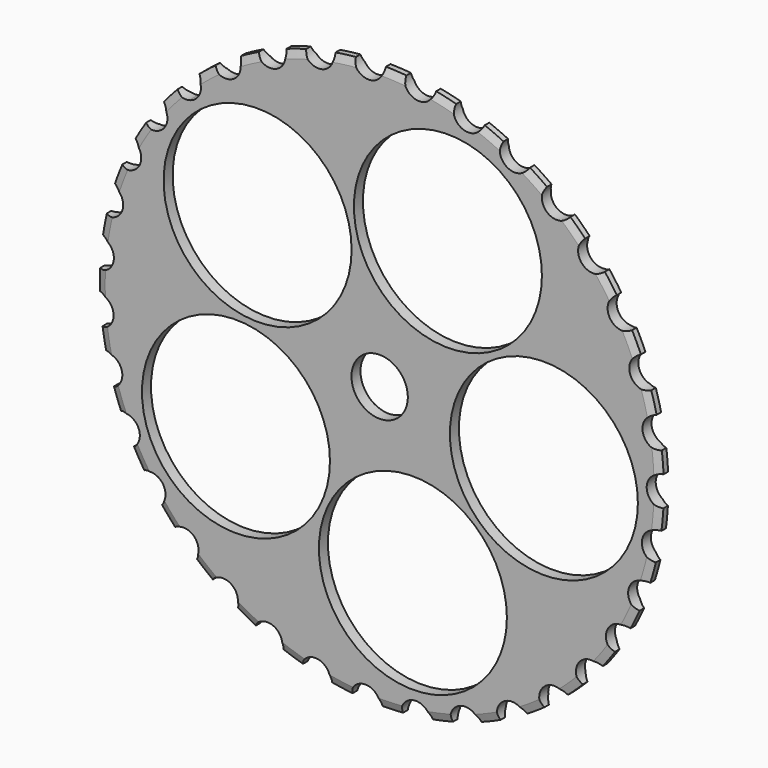
from build123d import *

# Parameters (mm, degrees)
F0_R     = 75
F0_R_2   = 25
F1_DEPTH = 3
F2_SIZE2 = 2
F2_SIZE  = 0.75
F4_R     = 4
F4_R_2   = 7.5
F5_DEPTH = 3.001


# Not quite as in the source:
# - two fillets or chamfers of one size are made in one step


with BuildPart() as f1:
    # F0 (on Front) → F1 (new body)
    with BuildSketch(Plane.XZ):
        Circle(F0_R)
        with Locations((-38.2195465563, -21.7165325156)):
            Circle(F0_R_2, mode=Mode.SUBTRACT)
        with Locations((8.8431603571, -43.0597264084)):
            Circle(F0_R_2, mode=Mode.SUBTRACT)
        with Locations((43.6849202249, -4.8958419511)):
            Circle(F0_R_2, mode=Mode.SUBTRACT)
        with Locations((-32.4641391635, 29.638171196)):
            Circle(F0_R_2, mode=Mode.SUBTRACT)
        with Locations((18.1556051377, 40.0339296791)):
            Circle(F0_R_2, mode=Mode.SUBTRACT)
    extrude(amount=F1_DEPTH)

    # F2
    f2_edges = [f1.edges().sort_by_distance(p)[0] for p in [
        (-75, 0, 0),
        (-75, -3, 0),
    ]]
    f2_side = f1.faces().sort_by_distance((-75, -1.5, 0))[0]
    chamfer(f2_edges, length=F2_SIZE, length2=F2_SIZE2, reference=f2_side)

    # F4 (on face) → F5 (cut, through all)
    with BuildSketch(Plane.XZ.offset(3)):
        with Locations((-67.4119440177, 32.9472917553)):
            Circle(F4_R)
        with Locations((-72.2115724518, 20.3809478261)):
            Circle(F4_R)
        with Locations((-74.6902615315, 7.1595434642)):
            Circle(F4_R)
        with Locations((-74.7683441501, -6.2919745154)):
            Circle(F4_R)
        with Locations((-72.4433106682, -19.5412632571)):
            Circle(F4_R)
        with Locations((-67.7898895749, -32.1624797191)):
            Circle(F4_R)
        with Locations((-60.9576456529, -43.7499676196)):
            Circle(F4_R)
        with Locations((-52.1661728435, -53.9312955632)):
            Circle(F4_R)
        with Locations((-41.6980363164, -62.3792272925)):
            Circle(F4_R)
        with Locations((-29.8896905929, -68.8222393309)):
            Circle(F4_R)
        with Locations((-17.1206656204, -73.05324797)):
            Circle(F4_R)
        with Locations((-3.8013683679, -74.936265111)):
            Circle(F4_R)
        with Locations((9.6401079917, -74.4107690336)):
            Circle(F4_R)
        with Locations((22.7717433485, -71.493649614)):
            Circle(F4_R)
        with Locations((35.1714761374, -66.2786654707)):
            Circle(F4_R)
        with Locations((46.4407687442, -58.9334304848)):
            Circle(F4_R)
        with Locations((56.2174168318, -49.6940265526)):
            Circle(F4_R)
        with Locations((64.1871908867, -38.8574157186)):
            Circle(F4_R)
        with Locations((70.0939358131, -26.7718955715)):
            Circle(F4_R)
        with Locations((73.7478039689, -13.8259046726)):
            Circle(F4_R)
        with Locations((75.0313570253, -0.4355378216)):
            Circle(F4_R)
        with Locations((73.9033405309, 12.9688275733)):
            Circle(F4_R)
        with Locations((70.400009864, 25.9563641793)):
            Circle(F4_R)
        with Locations((64.6339649547, 38.1096418835)):
            Circle(F4_R)
        with Locations((56.7905312308, 49.0380443409)):
            Circle(F4_R)
        with Locations((47.1218031057, 58.3903237046)):
            Circle(F4_R)
        with Locations((35.9385414568, 65.8658900207)):
            Circle(F4_R)
        with Locations((23.6001855152, 71.2244724368)):
            Circle(F4_R)
        with Locations((10.5033001928, 74.2938417052)):
            Circle(F4_R)
        with Locations((-2.9311698399, 74.975345772)):
            Circle(F4_R)
        with Locations((-16.2714296622, 73.2470805357)):
            Circle(F4_R)
        with Locations((-29.0887123469, 69.1645938632)):
            Circle(F4_R)
        with Locations((-40.9710598826, 62.859100235)):
            Circle(F4_R)
        with BuildLine():
            ThreePointArc((-50.6359663683, 50.6359663683), (-48.4058778237, 52.043523448), (-47.5365638425, 54.5332634047))
            ThreePointArc((-47.5365638425, 54.5332634047), (-51.0833465356, 58.5075047251), (-55.4338608789, 55.4338608789))
            Line((-55.4338608789, 55.4338608789), (-50.6359663683, 50.6359663683))
        make_face()
        with BuildLine():
            Line((-50.6359663683, 50.6359663683), (-55.4338608789, 55.4338608789))
            ThreePointArc((-55.4338608789, 55.4338608789), (-54.3649909673, 51.7048362799), (-50.6359663683, 50.6359663683))
        make_face()
        with Locations((-60.4456402361, 44.4546826184)):
            Circle(F4_R)
        Circle(F4_R_2)
    extrude(amount=-F5_DEPTH, mode=Mode.SUBTRACT)


solid = f1.part
